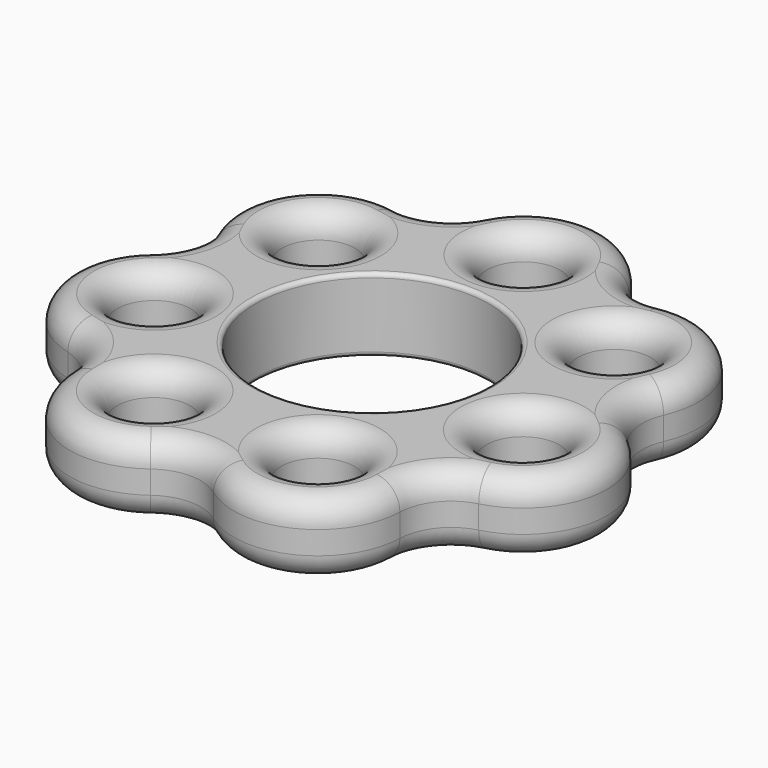
from build123d import *

# Parameters (mm, degrees)
F1_DEPTH     = 7
F2_R         = 11.125
F3_DEPTH     = 7.001
F4_R         = 3.5
F5_DEPTH     = 7.001
F6_R         = 0.4
F7_T2_ANGLE  = 73.8489971621
F7_T4_ANGLE  = 125.2775685907
F7_T6_ANGLE  = 125.2775685907
F7_T8_ANGLE  = 73.8489971621
F7_T10_ANGLE = 73.8489971621
F7_T12_ANGLE = 125.2775685907
F7_T14_ANGLE = 125.2775685907
F7_T16_ANGLE = 73.8489971621
F7_T18_ANGLE = 73.8489971621
F7_T20_ANGLE = 125.2775685907
F7_T22_ANGLE = 125.2775685907
F7_T24_ANGLE = 73.8489971621
F7_T26_ANGLE = 73.8489971621
F7_T28_ANGLE = 125.2775685907
F7_T44_ANGLE = 73.8489971621
F7_T46_ANGLE = 125.2775685907
F7_T48_ANGLE = 125.2775685907
F7_T50_ANGLE = 73.8489971621
F7_T52_ANGLE = 73.8489971621
F7_T54_ANGLE = 125.2775685907
F7_T56_ANGLE = 125.2775685907
F7_T58_ANGLE = 73.8489971621
F7_T60_ANGLE = 73.8489971621
F7_T62_ANGLE = 125.2775685907
F7_T64_ANGLE = 125.2775685907
F7_T66_ANGLE = 73.8489971621
F7_T68_ANGLE = 73.8489971621
F7_T70_ANGLE = 125.2775685907


# Not quite as in the source:
# - a fillet or chamfer that OpenCascade refuses, or shapes differently, is made with other operations: its cross-section is extruded or revolved along the edge and cut away or added


with BuildPart() as f1:
    # F0 (on Top) → F1 (new body)
    with BuildSketch(Plane.XY):
        with BuildLine():
            ThreePointArc((12.5176930718, 19.0701805763), (9.3762283683, 19.469938826), (7.1050135778, 21.6767896403))
            ThreePointArc((7.1050135778, 21.6767896403), (0, 26), (-7.1050135778, 21.6767896403))
            ThreePointArc((-7.1050135778, 21.6767896403), (-9.3762283683, 19.469938826), (-12.5176930718, 19.0701805763))
            ThreePointArc((-12.5176930718, 19.0701805763), (-20.3276185442, 16.2107348483), (-21.3775000875, 7.9603339793))
            ThreePointArc((-21.3775000875, 7.9603339793), (-21.0681939035, 4.8086777757), (-22.714321524, 2.1033365775))
            ThreePointArc((-22.714321524, 2.1033365775), (-25.3481257167, -5.7855442829), (-19.5522930097, -11.7504155294))
            ThreePointArc((-19.5522930097, -11.7504155294), (-16.8953797164, -13.4736157189), (-15.8066025808, -16.4473627644))
            ThreePointArc((-15.8066025808, -16.4473627644), (-11.2809772171, -23.4251905655), (-3.0038105016, -22.6128624796))
            ThreePointArc((-3.0038105016, -22.6128624796), (0, -21.6100017655), (3.0038105016, -22.6128624796))
            ThreePointArc((3.0038105016, -22.6128624796), (11.2809772171, -23.4251905655), (15.8066025808, -16.4473627644))
            ThreePointArc((15.8066025808, -16.4473627644), (16.8953797164, -13.4736157189), (19.5522930097, -11.7504155294))
            ThreePointArc((19.5522930097, -11.7504155294), (25.3481257167, -5.7855442829), (22.714321524, 2.1033365775))
            ThreePointArc((22.714321524, 2.1033365775), (21.0681939035, 4.8086777757), (21.3775000875, 7.9603339793))
            ThreePointArc((21.3775000875, 7.9603339793), (20.3276185442, 16.2107348483), (12.5176930718, 19.0701805763))
        make_face()
    extrude(amount=F1_DEPTH)

    # F2 (on face) → F3 (cut, through all)
    with BuildSketch(Plane.XY.offset(7)):
        Circle(F2_R)
    extrude(amount=-F3_DEPTH, mode=Mode.SUBTRACT)

    # F4 (on face) → F5 (cut, through all)
    with BuildSketch(Plane.XY.offset(7)):
        with Locations((0, 18)):
            Circle(F4_R)
        with Locations((-14.0729666844, 11.2228164335)):
            Circle(F4_R)
        with Locations((-17.5487024193, -4.0053768112)):
            Circle(F4_R)
        with Locations((-7.8099073041, -16.2174396222)):
            Circle(F4_R)
        with Locations((7.8099073041, -16.2174396222)):
            Circle(F4_R)
        with Locations((17.5487024193, -4.0053768112)):
            Circle(F4_R)
        with Locations((14.0729666844, 11.2228164335)):
            Circle(F4_R)
    extrude(amount=-F5_DEPTH, mode=Mode.SUBTRACT)

    # F6
    f6_edges = [f1.edges().sort_by_distance(p)[0] for p in [
        (-11.125, 0, 7),
        (11.125, 0, 3.5),
        (-11.125, 0, 0),
    ]]
    fillet(f6_edges, radius=F6_R)

    # F7: fillet of radius 2.4 on 44 edges, made by hand

    # F7_s1 → F7_t2 (revolve, cut)
    with BuildSketch(Plane(origin=(15.6812705957, 3.1078800379, 0), x_dir=(0, 0, 1), z_dir=(0.9809205179, 0.1944092016, 0))):
        with BuildLine():
            ThreePointArc((4.6, -16.2727766907), (6.2970562748, -15.5698329656), (7, -13.8727766907))
            Line((7, -13.8727766907), (7, -16.2727766907))
            Line((7, -16.2727766907), (4.6, -16.2727766907))
        make_face()
    revolve(axis=Axis((11.5456470639, 23.9747831655, 7), (0, 0, -1)), revolution_arc=F7_T2_ANGLE, mode=Mode.SUBTRACT)

    # F7_s3 → F7_t4 (revolve, cut)
    with BuildSketch(Plane(origin=(6.5193699752, 14.5965400336, 0), x_dir=(0, 0, 1), z_dir=(-0.4078103068, -0.9130666754, 0))):
        with BuildLine():
            ThreePointArc((4.6, -16.2727766907), (6.2970562748, -15.5698329656), (7, -13.8727766907))
            Line((7, -13.8727766907), (7, -16.2727766907))
            Line((7, -16.2727766907), (4.6, -16.2727766907))
        make_face()
    revolve(axis=Axis((14.0729666844, 11.2228164335, 7), (0, 0, 1)), revolution_arc=F7_T4_ANGLE, mode=Mode.SUBTRACT)

    # F7_s5 → F7_t6 (revolve, cut)
    with BuildSketch(Plane(origin=(-7.3472738392, 14.1978425458, 0), x_dir=(0, 0, 1), z_dir=(0.459598705, -0.8881266972, 0))):
        with BuildLine():
            ThreePointArc((4.6, -16.2727766907), (6.2970562748, -15.5698329656), (7, -13.8727766907))
            Line((7, -13.8727766907), (7, -16.2727766907))
            Line((7, -16.2727766907), (4.6, -16.2727766907))
        make_face()
    revolve(axis=Axis((0, 18, 7), (0, 0, 1)), revolution_arc=F7_T6_ANGLE, mode=Mode.SUBTRACT)

    # F7_s7 → F7_t8 (revolve, cut)
    with BuildSketch(Plane(origin=(12.206950754, -10.3223795278, 0), x_dir=(0, 0, 1), z_dir=(0.7635891736, -0.6457023881, 0))):
        with BuildLine():
            ThreePointArc((4.6, -16.2727766907), (6.2970562748, -15.5698329656), (7, -13.8727766907))
            Line((7, -13.8727766907), (7, -16.2727766907))
            Line((7, -16.2727766907), (4.6, -16.2727766907))
        make_face()
    revolve(axis=Axis((25.9428334644, 5.9212824454, 7), (0, 0, -1)), revolution_arc=F7_T8_ANGLE, mode=Mode.SUBTRACT)

    # F7_s9 → F7_t10 (revolve, cut)
    with BuildSketch(Plane(origin=(7.3472738392, 14.1978425458, 0), x_dir=(0, 0, 1), z_dir=(0.459598705, 0.8881266972, 0))):
        with BuildLine():
            ThreePointArc((4.6, -16.2727766907), (6.2970562748, -15.5698329656), (7, -13.8727766907))
            Line((7, -13.8727766907), (7, -16.2727766907))
            Line((7, -16.2727766907), (4.6, -16.2727766907))
        make_face()
    revolve(axis=Axis((-11.5456470639, 23.9747831655, 7), (0, 0, -1)), revolution_arc=F7_T10_ANGLE, mode=Mode.SUBTRACT)

    # F7_s11 → F7_t12 (revolve, cut)
    with BuildSketch(Plane(origin=(15.4767952274, 4.0037451608, 0), x_dir=(0, 0, 1), z_dir=(-0.9681298398, -0.2504488238, 0))):
        with BuildLine():
            ThreePointArc((4.6, -16.2727766907), (6.2970562748, -15.5698329656), (7, -13.8727766907))
            Line((7, -13.8727766907), (7, -16.2727766907))
            Line((7, -16.2727766907), (4.6, -16.2727766907))
        make_face()
    revolve(axis=Axis((17.5487024193, -4.0053768112, 7), (0, 0, 1)), revolution_arc=F7_T12_ANGLE, mode=Mode.SUBTRACT)

    # F7_s13 → F7_t14 (revolve, cut)
    with BuildSketch(Plane(origin=(-15.6812705957, 3.1078800379, 0), x_dir=(0, 0, 1), z_dir=(0.9809205179, -0.1944092016, 0))):
        with BuildLine():
            ThreePointArc((4.6, -16.2727766907), (6.2970562748, -15.5698329656), (7, -13.8727766907))
            Line((7, -13.8727766907), (7, -16.2727766907))
            Line((7, -16.2727766907), (4.6, -16.2727766907))
        make_face()
    revolve(axis=Axis((-14.0729666844, 11.2228164335, 7), (0, 0, 1)), revolution_arc=F7_T14_ANGLE, mode=Mode.SUBTRACT)

    # F7_s15 → F7_t16 (revolve, cut)
    with BuildSketch(Plane(origin=(-0.4594519819, -15.9796767709, 0), x_dir=(0, 0, 1), z_dir=(-0.0287403928, -0.9995869096, 0))):
        with BuildLine():
            ThreePointArc((4.6, -16.2727766907), (6.2970562748, -15.5698329656), (7, -13.8727766907))
            Line((7, -13.8727766907), (7, -16.2727766907))
            Line((7, -16.2727766907), (4.6, -16.2727766907))
        make_face()
    revolve(axis=Axis((20.8045371288, -16.5910647282, 7), (0, 0, -1)), revolution_arc=F7_T16_ANGLE, mode=Mode.SUBTRACT)

    # F7_s17 → F7_t18 (revolve, cut)
    with BuildSketch(Plane(origin=(-6.5193699752, 14.5965400336, 0), x_dir=(0, 0, 1), z_dir=(-0.4078103068, 0.9130666754, 0))):
        with BuildLine():
            ThreePointArc((4.6, -16.2727766907), (6.2970562748, -15.5698329656), (7, -13.8727766907))
            Line((7, -13.8727766907), (7, -16.2727766907))
            Line((7, -16.2727766907), (4.6, -16.2727766907))
        make_face()
    revolve(axis=Axis((-25.9428334644, 5.9212824454, 7), (0, 0, -1)), revolution_arc=F7_T18_ANGLE, mode=Mode.SUBTRACT)

    # F7_s19 → F7_t20 (revolve, cut)
    with BuildSketch(Plane(origin=(12.7798780043, -9.6039514795, 0), x_dir=(0, 0, 1), z_dir=(-0.7994278572, 0.6007621003, 0))):
        with BuildLine():
            ThreePointArc((4.6, -16.2727766907), (6.2970562748, -15.5698329656), (7, -13.8727766907))
            Line((7, -13.8727766907), (7, -16.2727766907))
            Line((7, -16.2727766907), (4.6, -16.2727766907))
        make_face()
    revolve(axis=Axis((7.8099073041, -16.2174396222, 7), (0, 0, 1)), revolution_arc=F7_T20_ANGLE, mode=Mode.SUBTRACT)

    # F7_s21 → F7_t22 (revolve, cut)
    with BuildSketch(Plane(origin=(-12.206950754, -10.3223795278, 0), x_dir=(0, 0, 1), z_dir=(0.7635891736, 0.6457023881, 0))):
        with BuildLine():
            ThreePointArc((4.6, -16.2727766907), (6.2970562748, -15.5698329656), (7, -13.8727766907))
            Line((7, -13.8727766907), (7, -16.2727766907))
            Line((7, -16.2727766907), (4.6, -16.2727766907))
        make_face()
    revolve(axis=Axis((-17.5487024193, -4.0053768112, 7), (0, 0, 1)), revolution_arc=F7_T22_ANGLE, mode=Mode.SUBTRACT)

    # F7_s23 → F7_t24 (revolve, cut)
    with BuildSketch(Plane(origin=(-12.7798780043, -9.6039514795, 0), x_dir=(0, 0, 1), z_dir=(-0.7994278572, -0.6007621003, 0))):
        with BuildLine():
            ThreePointArc((4.6, -16.2727766907), (6.2970562748, -15.5698329656), (7, -13.8727766907))
            Line((7, -13.8727766907), (7, -16.2727766907))
            Line((7, -16.2727766907), (4.6, -16.2727766907))
        make_face()
    revolve(axis=Axis((0, -26.6100017655, 7), (0, 0, -1)), revolution_arc=F7_T24_ANGLE, mode=Mode.SUBTRACT)

    # F7_s25 → F7_t26 (revolve, cut)
    with BuildSketch(Plane(origin=(-15.4767952274, 4.0037451608, 0), x_dir=(0, 0, 1), z_dir=(-0.9681298398, 0.2504488238, 0))):
        with BuildLine():
            ThreePointArc((4.6, -16.2727766907), (6.2970562748, -15.5698329656), (7, -13.8727766907))
            Line((7, -13.8727766907), (7, -16.2727766907))
            Line((7, -16.2727766907), (4.6, -16.2727766907))
        make_face()
    revolve(axis=Axis((-20.8045371288, -16.5910647282, 7), (0, 0, -1)), revolution_arc=F7_T26_ANGLE, mode=Mode.SUBTRACT)

    # F7_s27 → F7_t28 (revolve, cut)
    with BuildSketch(Plane(origin=(0.4594519819, -15.9796767709, 0), x_dir=(0, 0, 1), z_dir=(-0.0287403928, 0.9995869096, 0))):
        with BuildLine():
            ThreePointArc((4.6, -16.2727766907), (6.2970562748, -15.5698329656), (7, -13.8727766907))
            Line((7, -13.8727766907), (7, -16.2727766907))
            Line((7, -16.2727766907), (4.6, -16.2727766907))
        make_face()
    revolve(axis=Axis((-7.8099073041, -16.2174396222, 7), (0, 0, 1)), revolution_arc=F7_T28_ANGLE, mode=Mode.SUBTRACT)

    # F7_s29 → F7_t30 (revolve, cut)
    with BuildSketch(Plane.XZ.offset(16.2174396222)):
        with BuildLine():
            ThreePointArc((-4.3099073041, 4.6), (-3.606963579, 6.2970562748), (-1.9099073041, 7))
            Line((-1.9099073041, 7), (-4.3099073041, 7))
            Line((-4.3099073041, 7), (-4.3099073041, 4.6))
        make_face()
    revolve(axis=Axis((-7.8099073041, -16.2174396222, 7), (0, 0, 1)), mode=Mode.SUBTRACT)

    # F7_s31 → F7_t32 (revolve, cut)
    with BuildSketch(Plane.XZ.offset(4.0053768112)):
        with BuildLine():
            ThreePointArc((-14.0487024193, 4.6), (-13.3457586941, 6.2970562748), (-11.6487024193, 7))
            Line((-11.6487024193, 7), (-14.0487024193, 7))
            Line((-14.0487024193, 7), (-14.0487024193, 4.6))
        make_face()
    revolve(axis=Axis((-17.5487024193, -4.0053768112, 7), (0, 0, 1)), mode=Mode.SUBTRACT)

    # F7_s33 → F7_t34 (revolve, cut)
    with BuildSketch(Plane.XZ.offset(16.2174396222)):
        with BuildLine():
            ThreePointArc((11.3099073041, 4.6), (12.0128510293, 6.2970562748), (13.7099073041, 7))
            Line((13.7099073041, 7), (11.3099073041, 7))
            Line((11.3099073041, 7), (11.3099073041, 4.6))
        make_face()
    revolve(axis=Axis((7.8099073041, -16.2174396222, 7), (0, 0, 1)), mode=Mode.SUBTRACT)

    # F7_s35 → F7_t36 (revolve, cut)
    with BuildSketch(Plane.XZ.offset(4.0053768112)):
        with BuildLine():
            ThreePointArc((21.0487024193, 4.6), (21.7516461444, 6.2970562748), (23.4487024193, 7))
            Line((23.4487024193, 7), (21.0487024193, 7))
            Line((21.0487024193, 7), (21.0487024193, 4.6))
        make_face()
    revolve(axis=Axis((17.5487024193, -4.0053768112, 7), (0, 0, 1)), mode=Mode.SUBTRACT)

    # F7_s37 → F7_t38 (revolve, cut)
    with BuildSketch(Plane.XZ.offset(-11.2228164335)):
        with BuildLine():
            ThreePointArc((-10.5729666844, 4.6), (-9.8700229593, 6.2970562748), (-8.1729666844, 7))
            Line((-8.1729666844, 7), (-10.5729666844, 7))
            Line((-10.5729666844, 7), (-10.5729666844, 4.6))
        make_face()
    revolve(axis=Axis((-14.0729666844, 11.2228164335, 7), (0, 0, 1)), mode=Mode.SUBTRACT)

    # F7_s39 → F7_t40 (revolve, cut)
    with BuildSketch(Plane.XZ.offset(-18)):
        with BuildLine():
            ThreePointArc((3.5, 4.6), (4.2029437252, 6.2970562748), (5.9, 7))
            Line((5.9, 7), (3.5, 7))
            Line((3.5, 7), (3.5, 4.6))
        make_face()
    revolve(axis=Axis((0, 18, 7), (0, 0, 1)), mode=Mode.SUBTRACT)

    # F7_s41 → F7_t42 (revolve, cut)
    with BuildSketch(Plane.XZ.offset(-11.2228164335)):
        with BuildLine():
            ThreePointArc((17.5729666844, 4.6), (18.2759104096, 6.2970562748), (19.9729666844, 7))
            Line((19.9729666844, 7), (17.5729666844, 7))
            Line((17.5729666844, 7), (17.5729666844, 4.6))
        make_face()
    revolve(axis=Axis((14.0729666844, 11.2228164335, 7), (0, 0, 1)), mode=Mode.SUBTRACT)

    # F7_s43 → F7_t44 (revolve, cut)
    with BuildSketch(Plane(origin=(15.6812705957, 3.1078800379, 0), x_dir=(0, 0, 1), z_dir=(0.9809205179, 0.1944092016, 0))):
        with BuildLine():
            ThreePointArc((0, -13.8727766907), (0.7029437252, -15.5698329656), (2.4, -16.2727766907))
            Line((2.4, -16.2727766907), (0, -16.2727766907))
            Line((0, -16.2727766907), (0, -13.8727766907))
        make_face()
    revolve(axis=Axis((11.5456470639, 23.9747831655, 0), (0, 0, -1)), revolution_arc=F7_T44_ANGLE, mode=Mode.SUBTRACT)

    # F7_s45 → F7_t46 (revolve, cut)
    with BuildSketch(Plane(origin=(6.5193699752, 14.5965400336, 0), x_dir=(0, 0, 1), z_dir=(-0.4078103068, -0.9130666754, 0))):
        with BuildLine():
            ThreePointArc((0, -13.8727766907), (0.7029437252, -15.5698329656), (2.4, -16.2727766907))
            Line((2.4, -16.2727766907), (0, -16.2727766907))
            Line((0, -16.2727766907), (0, -13.8727766907))
        make_face()
    revolve(axis=Axis((14.0729666844, 11.2228164335, 0), (0, 0, 1)), revolution_arc=F7_T46_ANGLE, mode=Mode.SUBTRACT)

    # F7_s47 → F7_t48 (revolve, cut)
    with BuildSketch(Plane(origin=(-7.3472738392, 14.1978425458, 0), x_dir=(0, 0, 1), z_dir=(0.459598705, -0.8881266972, 0))):
        with BuildLine():
            ThreePointArc((0, -13.8727766907), (0.7029437252, -15.5698329656), (2.4, -16.2727766907))
            Line((2.4, -16.2727766907), (0, -16.2727766907))
            Line((0, -16.2727766907), (0, -13.8727766907))
        make_face()
    revolve(axis=Axis((0, 18, 0), (0, 0, 1)), revolution_arc=F7_T48_ANGLE, mode=Mode.SUBTRACT)

    # F7_s49 → F7_t50 (revolve, cut)
    with BuildSketch(Plane(origin=(12.206950754, -10.3223795278, 0), x_dir=(0, 0, 1), z_dir=(0.7635891736, -0.6457023881, 0))):
        with BuildLine():
            ThreePointArc((0, -13.8727766907), (0.7029437252, -15.5698329656), (2.4, -16.2727766907))
            Line((2.4, -16.2727766907), (0, -16.2727766907))
            Line((0, -16.2727766907), (0, -13.8727766907))
        make_face()
    revolve(axis=Axis((25.9428334644, 5.9212824454, 0), (0, 0, -1)), revolution_arc=F7_T50_ANGLE, mode=Mode.SUBTRACT)

    # F7_s51 → F7_t52 (revolve, cut)
    with BuildSketch(Plane(origin=(7.3472738392, 14.1978425458, 0), x_dir=(0, 0, 1), z_dir=(0.459598705, 0.8881266972, 0))):
        with BuildLine():
            ThreePointArc((0, -13.8727766907), (0.7029437252, -15.5698329656), (2.4, -16.2727766907))
            Line((2.4, -16.2727766907), (0, -16.2727766907))
            Line((0, -16.2727766907), (0, -13.8727766907))
        make_face()
    revolve(axis=Axis((-11.5456470639, 23.9747831655, 0), (0, 0, -1)), revolution_arc=F7_T52_ANGLE, mode=Mode.SUBTRACT)

    # F7_s53 → F7_t54 (revolve, cut)
    with BuildSketch(Plane(origin=(15.4767952274, 4.0037451608, 0), x_dir=(0, 0, 1), z_dir=(-0.9681298398, -0.2504488238, 0))):
        with BuildLine():
            ThreePointArc((0, -13.8727766907), (0.7029437252, -15.5698329656), (2.4, -16.2727766907))
            Line((2.4, -16.2727766907), (0, -16.2727766907))
            Line((0, -16.2727766907), (0, -13.8727766907))
        make_face()
    revolve(axis=Axis((17.5487024193, -4.0053768112, 0), (0, 0, 1)), revolution_arc=F7_T54_ANGLE, mode=Mode.SUBTRACT)

    # F7_s55 → F7_t56 (revolve, cut)
    with BuildSketch(Plane(origin=(-15.6812705957, 3.1078800379, 0), x_dir=(0, 0, 1), z_dir=(0.9809205179, -0.1944092016, 0))):
        with BuildLine():
            ThreePointArc((0, -13.8727766907), (0.7029437252, -15.5698329656), (2.4, -16.2727766907))
            Line((2.4, -16.2727766907), (0, -16.2727766907))
            Line((0, -16.2727766907), (0, -13.8727766907))
        make_face()
    revolve(axis=Axis((-14.0729666844, 11.2228164335, 0), (0, 0, 1)), revolution_arc=F7_T56_ANGLE, mode=Mode.SUBTRACT)

    # F7_s57 → F7_t58 (revolve, cut)
    with BuildSketch(Plane(origin=(-0.4594519819, -15.9796767709, 0), x_dir=(0, 0, 1), z_dir=(-0.0287403928, -0.9995869096, 0))):
        with BuildLine():
            ThreePointArc((0, -13.8727766907), (0.7029437252, -15.5698329656), (2.4, -16.2727766907))
            Line((2.4, -16.2727766907), (0, -16.2727766907))
            Line((0, -16.2727766907), (0, -13.8727766907))
        make_face()
    revolve(axis=Axis((20.8045371288, -16.5910647282, 0), (0, 0, -1)), revolution_arc=F7_T58_ANGLE, mode=Mode.SUBTRACT)

    # F7_s59 → F7_t60 (revolve, cut)
    with BuildSketch(Plane(origin=(-6.5193699752, 14.5965400336, 0), x_dir=(0, 0, 1), z_dir=(-0.4078103068, 0.9130666754, 0))):
        with BuildLine():
            ThreePointArc((0, -13.8727766907), (0.7029437252, -15.5698329656), (2.4, -16.2727766907))
            Line((2.4, -16.2727766907), (0, -16.2727766907))
            Line((0, -16.2727766907), (0, -13.8727766907))
        make_face()
    revolve(axis=Axis((-25.9428334644, 5.9212824454, 0), (0, 0, -1)), revolution_arc=F7_T60_ANGLE, mode=Mode.SUBTRACT)

    # F7_s61 → F7_t62 (revolve, cut)
    with BuildSketch(Plane(origin=(12.7798780043, -9.6039514795, 0), x_dir=(0, 0, 1), z_dir=(-0.7994278572, 0.6007621003, 0))):
        with BuildLine():
            ThreePointArc((0, -13.8727766907), (0.7029437252, -15.5698329656), (2.4, -16.2727766907))
            Line((2.4, -16.2727766907), (0, -16.2727766907))
            Line((0, -16.2727766907), (0, -13.8727766907))
        make_face()
    revolve(axis=Axis((7.8099073041, -16.2174396222, 0), (0, 0, 1)), revolution_arc=F7_T62_ANGLE, mode=Mode.SUBTRACT)

    # F7_s63 → F7_t64 (revolve, cut)
    with BuildSketch(Plane(origin=(-12.206950754, -10.3223795278, 0), x_dir=(0, 0, 1), z_dir=(0.7635891736, 0.6457023881, 0))):
        with BuildLine():
            ThreePointArc((0, -13.8727766907), (0.7029437252, -15.5698329656), (2.4, -16.2727766907))
            Line((2.4, -16.2727766907), (0, -16.2727766907))
            Line((0, -16.2727766907), (0, -13.8727766907))
        make_face()
    revolve(axis=Axis((-17.5487024193, -4.0053768112, 0), (0, 0, 1)), revolution_arc=F7_T64_ANGLE, mode=Mode.SUBTRACT)

    # F7_s65 → F7_t66 (revolve, cut)
    with BuildSketch(Plane(origin=(-12.7798780043, -9.6039514795, 0), x_dir=(0, 0, 1), z_dir=(-0.7994278572, -0.6007621003, 0))):
        with BuildLine():
            ThreePointArc((0, -13.8727766907), (0.7029437252, -15.5698329656), (2.4, -16.2727766907))
            Line((2.4, -16.2727766907), (0, -16.2727766907))
            Line((0, -16.2727766907), (0, -13.8727766907))
        make_face()
    revolve(axis=Axis((0, -26.6100017655, 0), (0, 0, -1)), revolution_arc=F7_T66_ANGLE, mode=Mode.SUBTRACT)

    # F7_s67 → F7_t68 (revolve, cut)
    with BuildSketch(Plane(origin=(-15.4767952274, 4.0037451608, 0), x_dir=(0, 0, 1), z_dir=(-0.9681298398, 0.2504488238, 0))):
        with BuildLine():
            ThreePointArc((0, -13.8727766907), (0.7029437252, -15.5698329656), (2.4, -16.2727766907))
            Line((2.4, -16.2727766907), (0, -16.2727766907))
            Line((0, -16.2727766907), (0, -13.8727766907))
        make_face()
    revolve(axis=Axis((-20.8045371288, -16.5910647282, 0), (0, 0, -1)), revolution_arc=F7_T68_ANGLE, mode=Mode.SUBTRACT)

    # F7_s69 → F7_t70 (revolve, cut)
    with BuildSketch(Plane(origin=(0.4594519819, -15.9796767709, 0), x_dir=(0, 0, 1), z_dir=(-0.0287403928, 0.9995869096, 0))):
        with BuildLine():
            ThreePointArc((0, -13.8727766907), (0.7029437252, -15.5698329656), (2.4, -16.2727766907))
            Line((2.4, -16.2727766907), (0, -16.2727766907))
            Line((0, -16.2727766907), (0, -13.8727766907))
        make_face()
    revolve(axis=Axis((-7.8099073041, -16.2174396222, 0), (0, 0, 1)), revolution_arc=F7_T70_ANGLE, mode=Mode.SUBTRACT)

    # F7_s71 → F7_t72 (revolve, cut)
    with BuildSketch(Plane.XZ.offset(16.2174396222)):
        with BuildLine():
            ThreePointArc((-1.9099073041, 0), (-3.606963579, 0.7029437252), (-4.3099073041, 2.4))
            Line((-4.3099073041, 2.4), (-4.3099073041, 0))
            Line((-4.3099073041, 0), (-1.9099073041, 0))
        make_face()
    revolve(axis=Axis((-7.8099073041, -16.2174396222, 0), (0, 0, 1)), mode=Mode.SUBTRACT)

    # F7_s73 → F7_t74 (revolve, cut)
    with BuildSketch(Plane.XZ.offset(4.0053768112)):
        with BuildLine():
            ThreePointArc((-11.6487024193, 0), (-13.3457586941, 0.7029437252), (-14.0487024193, 2.4))
            Line((-14.0487024193, 2.4), (-14.0487024193, 0))
            Line((-14.0487024193, 0), (-11.6487024193, 0))
        make_face()
    revolve(axis=Axis((-17.5487024193, -4.0053768112, 0), (0, 0, 1)), mode=Mode.SUBTRACT)

    # F7_s75 → F7_t76 (revolve, cut)
    with BuildSketch(Plane.XZ.offset(16.2174396222)):
        with BuildLine():
            ThreePointArc((13.7099073041, 0), (12.0128510293, 0.7029437252), (11.3099073041, 2.4))
            Line((11.3099073041, 2.4), (11.3099073041, 0))
            Line((11.3099073041, 0), (13.7099073041, 0))
        make_face()
    revolve(axis=Axis((7.8099073041, -16.2174396222, 0), (0, 0, 1)), mode=Mode.SUBTRACT)

    # F7_s77 → F7_t78 (revolve, cut)
    with BuildSketch(Plane.XZ.offset(4.0053768112)):
        with BuildLine():
            ThreePointArc((23.4487024193, 0), (21.7516461444, 0.7029437252), (21.0487024193, 2.4))
            Line((21.0487024193, 2.4), (21.0487024193, 0))
            Line((21.0487024193, 0), (23.4487024193, 0))
        make_face()
    revolve(axis=Axis((17.5487024193, -4.0053768112, 0), (0, 0, 1)), mode=Mode.SUBTRACT)

    # F7_s79 → F7_t80 (revolve, cut)
    with BuildSketch(Plane.XZ.offset(-11.2228164335)):
        with BuildLine():
            ThreePointArc((-8.1729666844, 0), (-9.8700229593, 0.7029437252), (-10.5729666844, 2.4))
            Line((-10.5729666844, 2.4), (-10.5729666844, 0))
            Line((-10.5729666844, 0), (-8.1729666844, 0))
        make_face()
    revolve(axis=Axis((-14.0729666844, 11.2228164335, 0), (0, 0, 1)), mode=Mode.SUBTRACT)

    # F7_s81 → F7_t82 (revolve, cut)
    with BuildSketch(Plane.XZ.offset(-18)):
        with BuildLine():
            ThreePointArc((5.9, 0), (4.2029437252, 0.7029437252), (3.5, 2.4))
            Line((3.5, 2.4), (3.5, 0))
            Line((3.5, 0), (5.9, 0))
        make_face()
    revolve(axis=Axis((0, 18, 0), (0, 0, 1)), mode=Mode.SUBTRACT)

    # F7_s83 → F7_t84 (revolve, cut)
    with BuildSketch(Plane.XZ.offset(-11.2228164335)):
        with BuildLine():
            ThreePointArc((19.9729666844, 0), (18.2759104096, 0.7029437252), (17.5729666844, 2.4))
            Line((17.5729666844, 2.4), (17.5729666844, 0))
            Line((17.5729666844, 0), (19.9729666844, 0))
        make_face()
    revolve(axis=Axis((14.0729666844, 11.2228164335, 0), (0, 0, 1)), mode=Mode.SUBTRACT)


solid = f1.part
